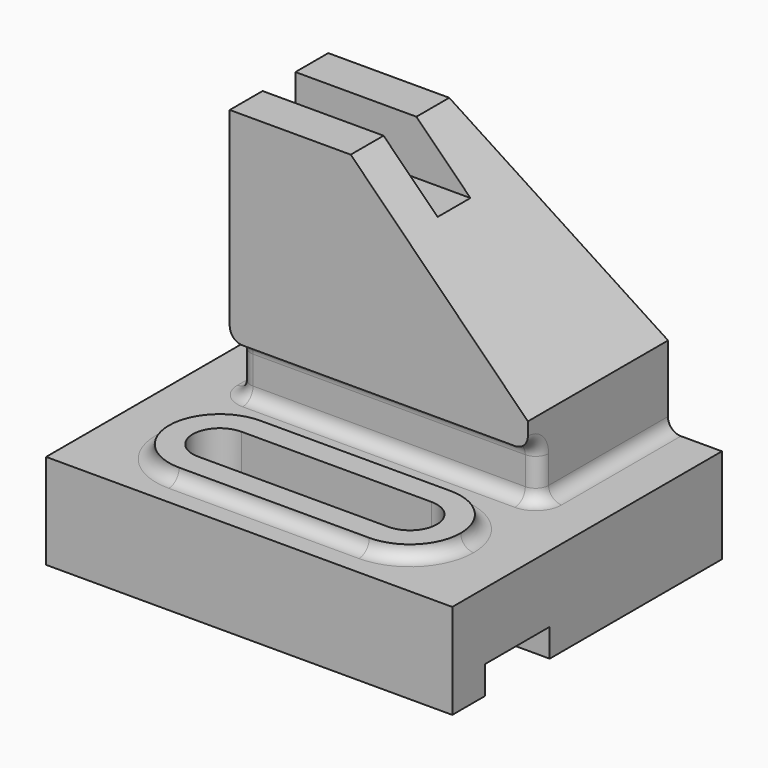
from build123d import *

# Parameters (mm, degrees)
F1_DEPTH = 95.504
F3_DEPTH = 3.048
F4_DEPTH = 22.353
F6_DEPTH = 41.148
F5_W     = 70.104
F5_H     = 12.7
F7_DEPTH = 38.1
F8_W     = 9.652
F8_H     = 12.7
F9_DEPTH = 82.805
F10_F1_R = 3.0479
F10_F2_R = 3.048
F10_F3_R = 3.048


# Not quite as in the source:
# - a fillet or chamfer is up to 0.001 mm smaller than in the source, because OpenCascade refuses the exact size


with BuildPart() as f1:
    # F0 (on Right) → F1 (new body)
    with BuildSketch(Plane.YZ):
        Polygon((39.624, -11.176), (39.624, 11.176), (-39.624, 11.176), (-39.624, -11.176), (-29.972, -11.176), (-29.972, -4.572), (-10.9982, -4.572), (-10.9982, -11.176), align=None)
    extrude(amount=F1_DEPTH)

    # F2 (on face) → F3 (join)
    with BuildSketch(Plane.XY.offset(11.176)):
        with BuildLine():
            ThreePointArc((25.4, -26.67), (19.05, -20.32), (25.4, -13.97))
            Line((25.4, -13.97), (35.509072361, -13.97))
            ThreePointArc((35.509072361, -13.97), (31.1753590365, -9.871982389), (25.4, -8.382))
            ThreePointArc((25.4, -8.382), (13.462, -20.32), (25.4, -32.258))
            ThreePointArc((25.4, -32.258), (31.1753590365, -30.768017611), (35.509072361, -26.67))
            Line((35.509072361, -26.67), (25.4, -26.67))
        make_face()
        with BuildLine():
            ThreePointArc((25.4, -8.382), (31.1753590365, -9.871982389), (35.509072361, -13.97))
            Line((35.509072361, -13.97), (59.994927639, -13.97))
            ThreePointArc((59.994927639, -13.97), (64.3286409635, -9.871982389), (70.104, -8.382))
            Line((70.104, -8.382), (25.4, -8.382))
        make_face()
        with BuildLine():
            Line((59.994927639, -26.67), (35.509072361, -26.67))
            ThreePointArc((35.509072361, -26.67), (31.1753590365, -30.768017611), (25.4, -32.258))
            Line((25.4, -32.258), (70.104, -32.258))
            ThreePointArc((70.104, -32.258), (64.3286409635, -30.768017611), (59.994927639, -26.67))
        make_face()
        with BuildLine():
            ThreePointArc((70.104, -8.382), (64.3286409635, -9.871982389), (59.994927639, -13.97))
            Line((59.994927639, -13.97), (70.104, -13.97))
            ThreePointArc((70.104, -13.97), (74.5941280605, -15.8298719395), (76.454, -20.32))
            ThreePointArc((76.454, -20.32), (74.5941280605, -24.8101280605), (70.104, -26.67))
            Line((70.104, -26.67), (59.994927639, -26.67))
            ThreePointArc((59.994927639, -26.67), (64.3286409635, -30.768017611), (70.104, -32.258))
            ThreePointArc((70.104, -32.258), (78.5454407538, -28.7614407538), (82.042, -20.32))
            ThreePointArc((82.042, -20.32), (78.5454407538, -11.8785592462), (70.104, -8.382))
        make_face()
    extrude(amount=F3_DEPTH)

    # F2 (on face) → F4 (cut, through all)
    with BuildSketch(Plane.XY.offset(11.176)):
        with BuildLine():
            ThreePointArc((25.4, -26.67), (29.8901280605, -24.8101280605), (31.75, -20.32))
            ThreePointArc((31.75, -20.32), (29.8901280605, -15.8298719395), (25.4, -13.97))
            ThreePointArc((25.4, -13.97), (19.05, -20.32), (25.4, -26.67))
        make_face()
        with BuildLine():
            ThreePointArc((25.4, -13.97), (29.8901280605, -15.8298719395), (31.75, -20.32))
            ThreePointArc((31.75, -20.32), (29.8901280605, -24.8101280605), (25.4, -26.67))
            Line((25.4, -26.67), (35.509072361, -26.67))
            ThreePointArc((35.509072361, -26.67), (36.8716596412, -23.6240685642), (37.338, -20.32))
            ThreePointArc((37.338, -20.32), (36.8716596412, -17.0159314358), (35.509072361, -13.97))
            Line((35.509072361, -13.97), (25.4, -13.97))
        make_face()
        with BuildLine():
            Line((59.994927639, -13.97), (35.509072361, -13.97))
            ThreePointArc((35.509072361, -13.97), (36.8716596412, -17.0159314358), (37.338, -20.32))
            ThreePointArc((37.338, -20.32), (36.8716596412, -23.6240685642), (35.509072361, -26.67))
            Line((35.509072361, -26.67), (59.994927639, -26.67))
            ThreePointArc((59.994927639, -26.67), (58.166, -20.32), (59.994927639, -13.97))
        make_face()
        with BuildLine():
            Line((70.104, -13.97), (59.994927639, -13.97))
            ThreePointArc((59.994927639, -13.97), (58.166, -20.32), (59.994927639, -26.67))
            Line((59.994927639, -26.67), (70.104, -26.67))
            ThreePointArc((70.104, -26.67), (63.754, -20.32), (70.104, -13.97))
        make_face()
        with BuildLine():
            ThreePointArc((76.454, -20.32), (74.5941280605, -15.8298719395), (70.104, -13.97))
            ThreePointArc((70.104, -13.97), (63.754, -20.32), (70.104, -26.67))
            ThreePointArc((70.104, -26.67), (74.5941280605, -24.8101280605), (76.454, -20.32))
        make_face()
    extrude(amount=-F4_DEPTH, mode=Mode.SUBTRACT)



with BuildPart() as f6:
    # F5 (on face) → F6 (new body)
    with BuildSketch(Plane(origin=(0, 39.624, 0), x_dir=(-1, 0, 0), z_dir=(0, 1, 0))):
        Polygon((-82.804, 29.972), (-82.804, 23.876), (-12.7, 23.876), (-12.7, 71.628), (-41.148, 71.628), align=None)
    extrude(amount=-F6_DEPTH)


with BuildPart() as f1_1:
    add(f1.part)

    add(f6.part)  # F7 merges F6
    # F5 (on face) → F7 (join)
    with BuildSketch(Plane(origin=(0, 39.624, 0), x_dir=(-1, 0, 0), z_dir=(0, 1, 0))):
        with Locations((-47.752, 17.526)):
            Rectangle(F5_W, F5_H)
    extrude(amount=-F7_DEPTH)

    # F8 (on face) → F9 (cut, through all)
    with BuildSketch(Plane(origin=(12.7, 0, 0), x_dir=(0, -1, 0), z_dir=(-1, 0, 0))):
        Polygon((-39.624, 71.628), (-39.624, 30.1498), (-27.432, 71.628), align=None)
        with Locations((-12.954, 65.278)):
            Rectangle(F8_W, F8_H)
    extrude(amount=-F9_DEPTH, mode=Mode.SUBTRACT)

    # F10: fillet of radius 3.048 on 10 edges, made by hand

    # F10_f1 (radius 3.048 in the source; OpenCascade refuses exactly that, so slightly less here)
    f10_f1_edges = [f1_1.edges().sort_by_distance(p)[0] for p in [
        (47.752, 1.524, 23.876),
        (47.752, -32.258, 11.176),
        (82.042, -20.32, 11.176),
        (47.752, -8.382, 11.176),
        (13.462, -20.32, 11.176),
    ]]
    fillet(f10_f1_edges, radius=F10_F1_R)

    # F10_f2
    f10_f2_edges = [f1_1.edges().sort_by_distance(p)[0] for p in [
        (82.804, 1.524, 16.00205),
        (12.7, 1.524, 16.00205),
        (12.7, 0.6312907584, 22.9832907584),
        (82.804, 0.6312907584, 22.9832907584),
    ]]
    fillet(f10_f2_edges, radius=F10_F2_R)

    # F10_f3
    f10_f3_edges = [f1_1.edges().sort_by_distance(p)[0] for p in [
        (47.752, 1.524, 11.176),
        (12.7, 22.098, 11.176),
        (82.804, 22.098, 11.176),
        (81.9112614691, 2.4167385309, 11.176),
        (13.5927385309, 2.4167385309, 11.176),
    ]]
    fillet(f10_f3_edges, radius=F10_F3_R)


solid = f1_1.part
